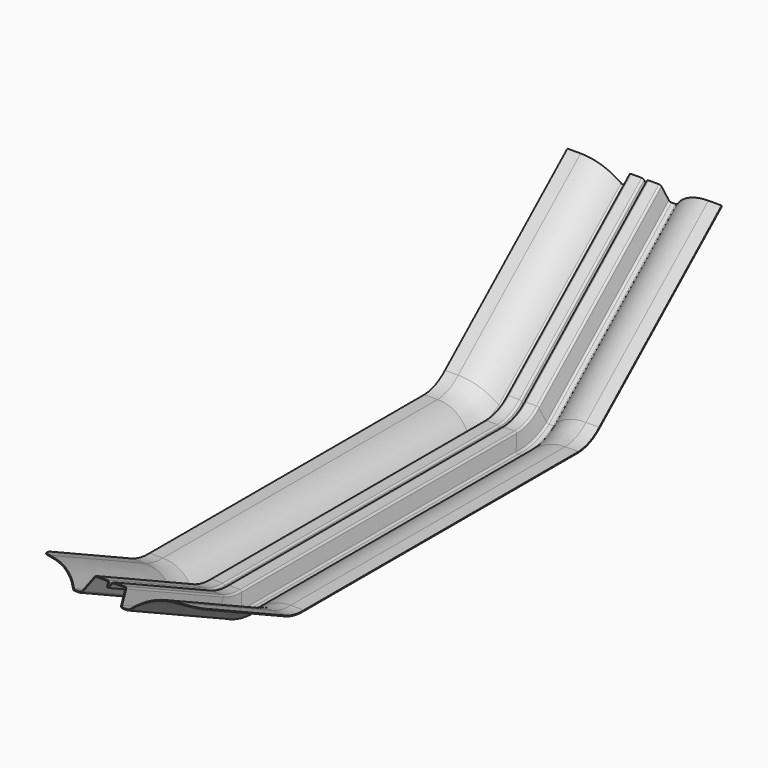
from build123d import *

# Parameters (mm, degrees)
F3_T1_DEPTH = 100.7999998219


# Not quite as in the source:
# - a fillet or chamfer that OpenCascade refuses, or shapes differently, is made with other operations: its cross-section is extruded or revolved along the edge and cut away or added


with BuildPart() as f2:
    # F2: sweep along a path in F1
    with BuildLine(Plane.YZ) as f2_path:
        Line((150, 130.3930106724), (11.2869739802, 9.8116167911))
        ThreePointArc((11.2869739802, 9.8116167911), (-0.947091929, 2.5331124301), (-14.9553871794, 0))
        Line((-14.9553871794, 0), (-326.2054046659, 0))
        ThreePointArc((-326.2054046659, 0), (-337.0273853629, 1.185199644), (-347.336317753, 4.6846106482))
        Line((-347.336317753, 4.6846106482), (-457.2901377981, 55.9569189786))
    # F0 (on Front) → F2 (sweep)
    with BuildSketch(Plane.XZ):
        with BuildLine():
            Line((-0.7626034073, -0.2417348926), (0, 0))
            Line((0, 0), (-1.14252585, 3.604337366))
            ThreePointArc((-1.14252585, 3.604337366), (-1.8676531294, 4.6137959493), (-3.0490347926, 5))
            Line((-3.0490347926, 5), (-12.5863364321, 5))
            ThreePointArc((-12.5863364321, 5), (-13.7893900926, 4.597705195), (-14.5084615153, 3.55266189))
            Line((-14.5084615153, 3.55266189), (-17.9890628447, -8.55266189))
            ThreePointArc((-17.9890628447, -8.55266189), (-18.7081342674, -9.597705195), (-19.9111879279, -10))
            Line((-19.9111879279, -10), (-23.7941965471, -10))
            ThreePointArc((-23.7941965471, -10), (-24.6857884236, -9.7902692328), (-25.3903860517, -9.2050639258))
            ThreePointArc((-25.3903860517, -9.2050639258), (-39.7538675659, 2.7245612566), (-57.929295532, 7))
            Line((-57.929295532, 7), (-69.929295532, 7))
            Line((-69.929295532, 7), (-69.929295532, 6.2000001781))
            Line((-69.929295532, 6.2000001781), (-57.929295532, 6.2000001781))
            ThreePointArc((-57.929295532, 6.2000001781), (-40.1105042371, 2.0084537229), (-26.0288617115, -9.6870893889))
            ThreePointArc((-26.0288617115, -9.6870893889), (-25.0424250948, -10.5063767665), (-23.7941965471, -10.7999998219))
            Line((-23.7941965471, -10.7999998219), (-19.9111879279, -10.7999998219))
            ThreePointArc((-19.9111879279, -10.7999998219), (-18.2269129103, -10.2367871307), (-17.2202129826, -8.7737265968))
            Line((-17.2202129826, -8.7737265968), (-13.7396116531, 3.3315971832))
            ThreePointArc((-13.7396116531, 3.3315971832), (-13.3081687355, 3.9586232592), (-12.5863364321, 4.2000001781))
            Line((-12.5863364321, 4.2000001781), (-3.0490347926, 4.2000001781))
            ThreePointArc((-3.0490347926, 4.2000001781), (-2.3402056895, 3.9682777133), (-1.9051292573, 3.3626024734))
            Line((-1.9051292573, 3.3626024734), (-0.7626034073, -0.2417348926))
        make_face()
    sweep(path=f2_path.line)

    # F3: fillet of radius 20 on 1 edges, made by hand

    # F3_s2 → F3_t1 (cut)
    with BuildSketch(Plane(origin=(0, -176.7893108528, -165.1161938842), x_dir=(1, 0, 0), z_dir=(0, -0.7308225533, -0.6825675026))):
        with BuildLine():
            ThreePointArc((-69.929295532, 333.0259657329), (-64.0714311557, 347.1681013567), (-49.929295532, 353.0259657329))
            Line((-49.929295532, 353.0259657329), (-69.929295532, 353.0259657329))
            Line((-69.929295532, 353.0259657329), (-69.929295532, 333.0259657329))
        make_face()
    extrude(amount=F3_T1_DEPTH, mode=Mode.SUBTRACT)

    # F4: F2 across plane


with BuildPart() as f2_1:
    add(f2.part)
    add(f2.part.mirror(Plane.YZ))


solid = f2_1.part
